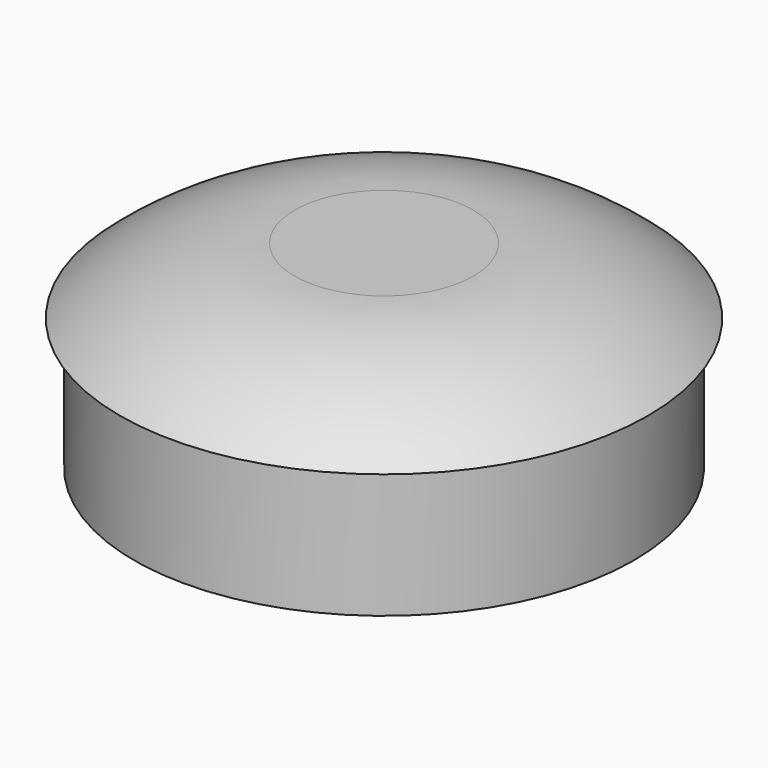
from build123d import *

# Parameters (mm, degrees)
F0_R     = 11.35
F0_R_2   = 10.9231311618
F1_DEPTH = 6
F0_R_3   = 12
F2_DEPTH = 3


# Not quite as in the source:
# - a fillet or chamfer that OpenCascade refuses, or shapes differently, is made with other operations: its cross-section is extruded or revolved along the edge and cut away or added


with BuildPart() as f1:
    # F0 (on Top) → F1 (new body)
    with BuildSketch(Plane.XY):
        Circle(F0_R)
        Circle(F0_R_2, mode=Mode.SUBTRACT)
    extrude(amount=-F1_DEPTH)

    # F0 (on Top) → F2 (join)
    with BuildSketch(Plane.XY):
        Circle(F0_R_3)
        Circle(F0_R, mode=Mode.SUBTRACT)
        Circle(F0_R)
        Circle(F0_R_2, mode=Mode.SUBTRACT)
        Circle(F0_R_2)
    extrude(amount=F2_DEPTH)

    # F3: fillet of radius 12 on 1 edges, made by hand

    # F3_s1 → F3_t2 (revolve, cut)
    with BuildSketch(Plane.XZ):
        with BuildLine():
            ThreePointArc((12, 0), (8.3053867539, 2.2249721603), (4.0627460668, 3))
            Line((4.0627460668, 3), (4.0627460668, 3.24))
            Line((4.0627460668, 3.24), (12, 3.24))
            Line((12, 3.24), (12.24, 3))
            ThreePointArc((12.24, 3), (12.24, 1.5), (12.1587450787, 0.18))
            Line((12.1587450787, 0.18), (12, 0))
        make_face()
    revolve(axis=Axis((0, 0, 3), (0, 0, 1)), mode=Mode.SUBTRACT)


solid = f1.part
